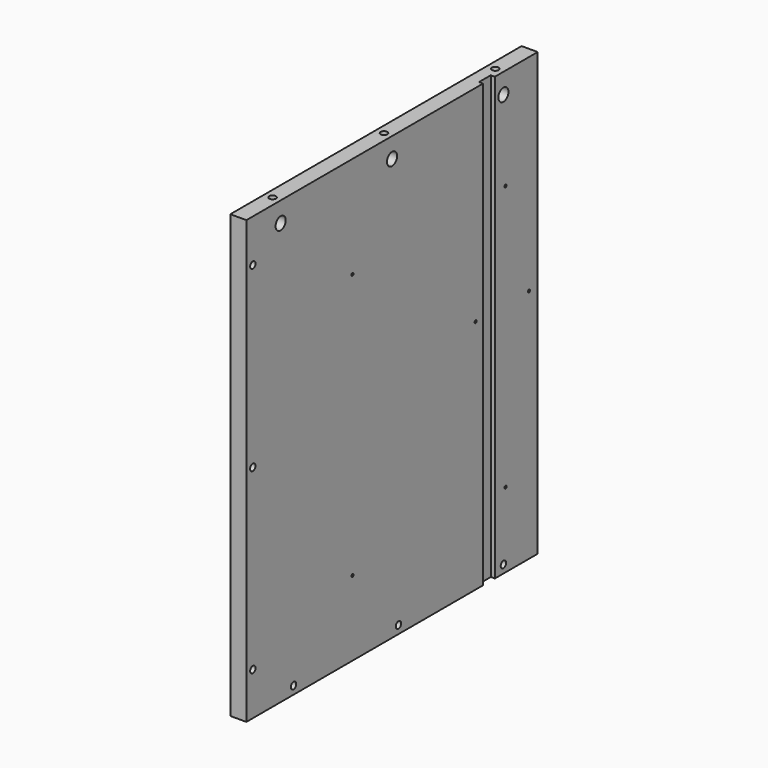
from build123d import *

# Parameters (mm, degrees)
F0_W      = 431.8
F0_H      = 523.875
F1_DEPTH  = 19.05
F3_D      = 8.001
F3_DEPTH  = 14.224
F3_TIP    = 2.4037429064
F4_D      = 15.0114
F4_DEPTH  = 14.224
F4_TIP    = 4.5098795482
F6_D      = 8.001
F6_DEPTH  = 25.4
F6_TIP    = 2.4037429064
F8_D      = 3.175
F8_DEPTH  = 14.224
F8_TIP    = 0.9538662327
F9_W      = 17.526
F9_H      = 523.875
F10_DEPTH = 4.826


with BuildPart() as f1:
    # F0 (on Right) → F1 (new body)
    with BuildSketch(Plane.YZ):
        Rectangle(F0_W, F0_H)
    extrude(amount=F1_DEPTH)

    # F3
    with Locations(Plane.YZ.offset(19.05)):
        with Locations((-206.375, 211.1375), (-206.375, 0), (-206.375, -211.1375), (-146.05, -252.4125), (9.525, -252.4125), (165.1, -252.4125)):
            Hole(F3_D / 2, depth=F3_DEPTH)
            with Locations((0, 0, -(F3_DEPTH + F3_TIP / 2))):  # 118° drill point
                Cone(0, F3_D / 2, F3_TIP, mode=Mode.SUBTRACT)

    # F4
    with Locations(Plane.YZ.offset(19.05)):
        with Locations((-165.1, 238.0615), (0, 238.0615), (165.1, 238.0615)):
            Hole(F4_D / 2, depth=F4_DEPTH)
            with Locations((0, 0, -(F4_DEPTH + F4_TIP / 2))):  # 118° drill point
                Cone(0, F4_D / 2, F4_TIP, mode=Mode.SUBTRACT)

    # F6
    with Locations(Plane.XY.offset(261.9375)):
        with Locations((9.525, 165.1), (9.525, 0), (9.525, -165.1)):
            Hole(F6_D / 2, depth=F6_DEPTH)
            with Locations((0, 0, -(F6_DEPTH + F6_TIP / 2))):  # 118° drill point
                Cone(0, F6_D / 2, F6_TIP, mode=Mode.SUBTRACT)

    # F8
    with Locations(Plane.YZ.offset(19.05)):
        with Locations((-58.7375, 141.4145), (168.275, 141.4145), (123.825, 17.7165), (203.2, 17.7165), (168.275, -173.0375), (-58.7375, -173.0375)):
            Hole(F8_D / 2, depth=F8_DEPTH)
            with Locations((0, 0, -(F8_DEPTH + F8_TIP / 2))):  # 118° drill point
                Cone(0, F8_D / 2, F8_TIP, mode=Mode.SUBTRACT)

    # F9 (on face) → F10 (cut)
    with BuildSketch(Plane.YZ.offset(19.05)):
        with Locations((143.637, 0)):
            Rectangle(F9_W, F9_H)
    extrude(amount=-F10_DEPTH, mode=Mode.SUBTRACT)


solid = f1.part
